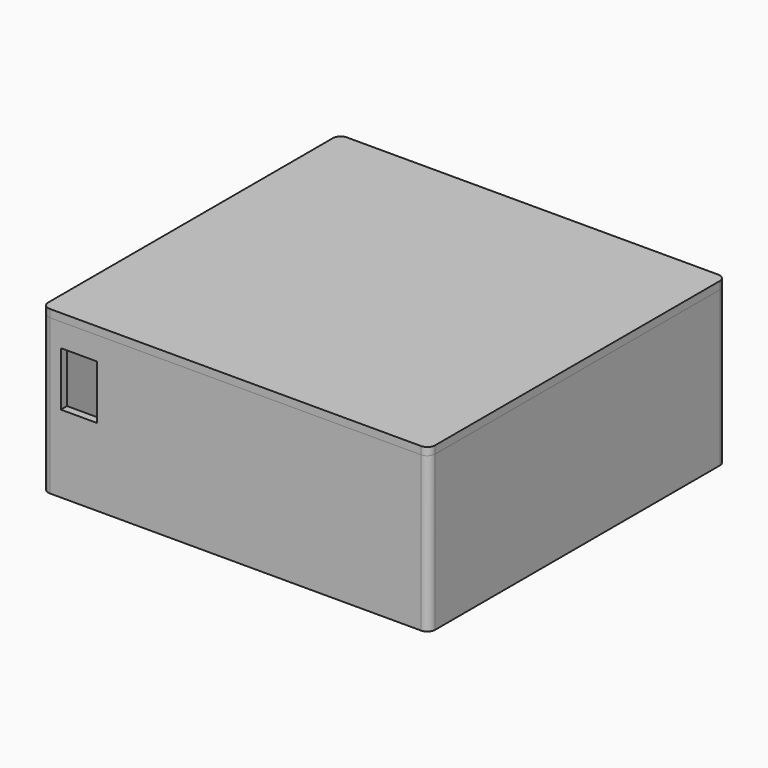
from build123d import *

# Parameters (mm, degrees)
F0_W      = 100
F0_H      = 96
F1_DEPTH  = 40
F2_T      = -2
F3_W      = 9.3
F3_H      = 14
F4_DEPTH  = 2
F5_W      = 2
F5_H      = 12
F5_H_2    = 16
F6_DEPTH  = 5
F7_R      = 2
F9_W      = 100
F9_H      = 96
F10_DEPTH = 2
F8_W      = 94.5
F8_H      = 90.5
F8_W_2    = 91.5
F8_H_2    = 87.5
F11_DEPTH = 2
F12_R     = 2


# Not quite as in the source:
# - a feature names something its author has since deleted; it is built from what else it names


with BuildPart() as f1:
    # F0 (on Top) → F1 (new body)
    with BuildSketch(Plane.XY):
        Rectangle(F0_W, F0_H)
    extrude(amount=F1_DEPTH)

    # F2
    f2_openings = [f1.faces().sort_by_distance(p)[0] for p in [
        (0, 0, 40),
    ]]
    offset(amount=F2_T, openings=f2_openings)

    # F3 (on face) → F4 (cut, through all)
    with BuildSketch(Plane.XZ.offset(48)):
        with Locations((-40.5, 27)):
            Rectangle(F3_W, F3_H)
    extrude(amount=-F4_DEPTH, mode=Mode.SUBTRACT)

    # F5 (on face) → F6 (join)
    with BuildSketch(Plane(origin=(0, 0, 0), x_dir=(1, 0, 0), z_dir=(0, 0, -1))):
        with Locations((-33, 32)):
            Rectangle(F5_W, F5_H)
        with Locations((-33, 0)):
            Rectangle(F5_W, F5_H_2)
        with Locations((-33, -32)):
            Rectangle(F5_W, F5_H)
    extrude(amount=-F6_DEPTH)

    # F7
    f7_edges = [f1.edges().sort_by_distance(p)[0] for p in [
        (-50, -48, 20),
        (50, -48, 20),
        (50, 48, 20),
        (-50, 48, 20),
    ]]
    fillet(f7_edges, radius=F7_R)


with BuildPart() as f10:
    # F9 (on face) → F10 (new body)
    with BuildSketch(Plane.XY.offset(40)):
        Rectangle(F9_W, F9_H)
    extrude(amount=F10_DEPTH)

    # F8 (on face) → F11 (join)
    with BuildSketch(Plane.XY.offset(40)):
        Rectangle(F8_W, F8_H)
        Rectangle(F8_W_2, F8_H_2, mode=Mode.SUBTRACT)
    extrude(amount=-F11_DEPTH)

    # F12
    f12_edges = [f10.edges().sort_by_distance(p)[0] for p in [
        (-50, -48, 41),
        (50, -48, 41),
        (50, 48, 41),
        (-50, 48, 41),
    ]]
    fillet(f12_edges, radius=F12_R)


solid = Compound([f1.part, f10.part])
